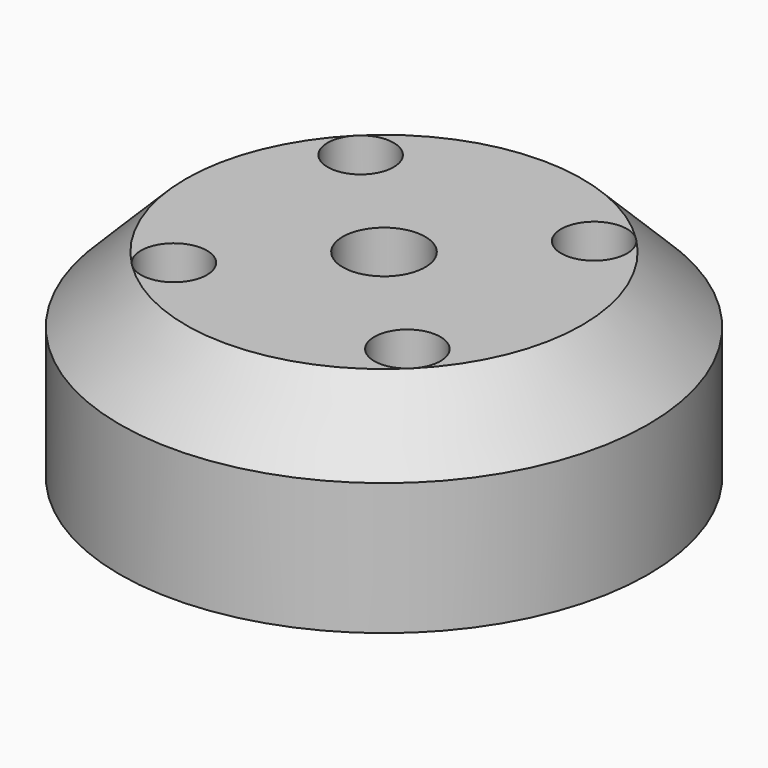
from build123d import *

# Parameters (mm, degrees)
F0_R     = 50.8
F1_DEPTH = 19.05
F2_SIZE  = 12.7
F4_D     = 12.7
F5_D     = 15.875


# Not quite as in the source:
# - a length typed as a fraction of an inch, garbled in the dataset ("3 / 203.2 mm" for 3/8 in), is restored


with BuildPart() as f1:
    # F0 (on Top) → F1 (new body, symmetric)
    with BuildSketch(Plane.XY):
        Circle(F0_R)
    extrude(amount=F1_DEPTH, both=True)

    # F2
    f2_edges = [f1.edges().sort_by_distance(p)[0] for p in [
        (-50.8, 0, 19.05),
    ]]
    chamfer(f2_edges, length=F2_SIZE)

    # F4 (through all)
    with Locations(Plane(origin=(0, 0, -19.05), x_dir=(1, 0, 0), z_dir=(0, 0, -1))):
        with Locations((-22.4506403027, 22.4506403027), (-22.4506403027, -22.4506403027), (22.4506403027, -22.4506403027), (22.4506403027, 22.4506403027)):
            Hole(F4_D / 2)

    # F5 (through all)
    with Locations(Plane(origin=(0, 0, -19.05), x_dir=(1, 0, 0), z_dir=(0, 0, -1))):
        with Locations((0, 0)):
            Hole(F5_D / 2)


solid = f1.part
